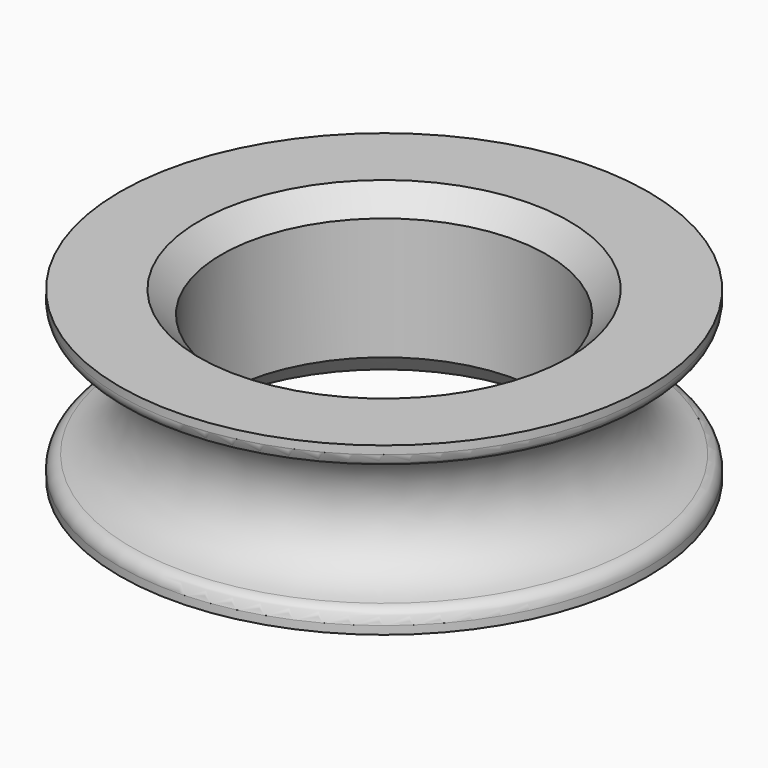
from build123d import *

# Parameters (mm, degrees)
F2_SIZE = 0.8


# Not quite as in the source:
# - a feature of the source that left no trace in its solid (it failed there, or was rolled back) is left out


with BuildPart() as f1:
    # F0 (on Front) → F1 (revolve)
    with BuildSketch(Plane.XZ):
        with BuildLine():
            Line((5.85, 6), (5.85, 0))
            Line((5.85, 0), (9.5, 0))
            Line((9.5, 0), (9.5, 0.294127265))
            ThreePointArc((9.5, 0.294127265), (9.3843349974, 0.6139500436), (9.090853561, 0.7858036122))
            ThreePointArc((9.090853561, 0.7858036122), (7.248319194, 3), (9.090853561, 5.2141963878))
            ThreePointArc((9.090853561, 5.2141963878), (9.3843349974, 5.3860499564), (9.5, 5.705872735))
            Line((9.5, 5.705872735), (9.5, 6))
            Line((9.5, 6), (5.85, 6))
        make_face()
    revolve(axis=Axis((0, 0, 22.371660918), (0, 0, 1)))

    # F2
    f2_edges = [f1.edges().sort_by_distance(p)[0] for p in [
        (-5.85, 0, 0),
        (-5.85, 0, 6),
    ]]
    chamfer(f2_edges, length=F2_SIZE)


solid = f1.part
